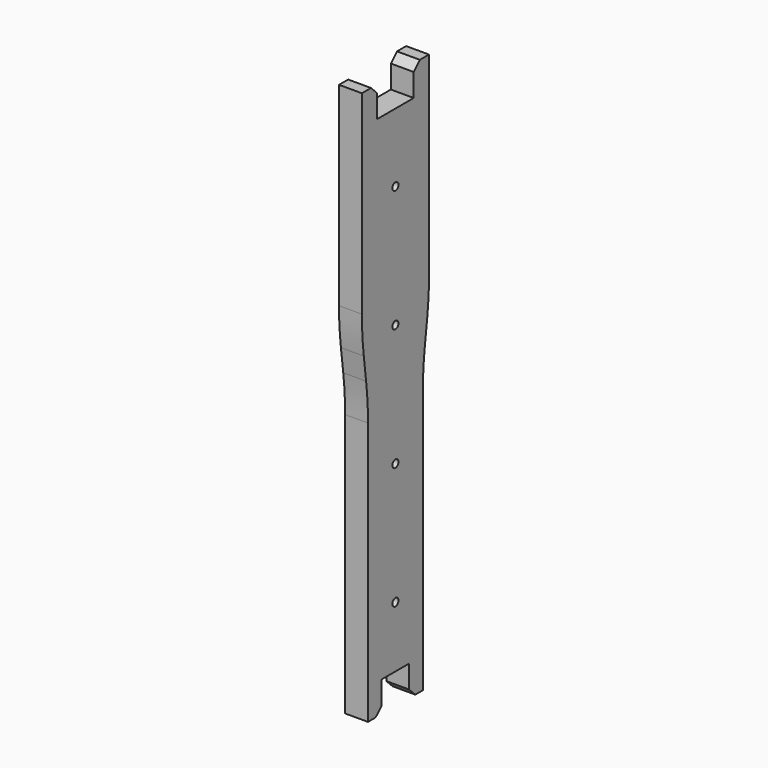
from build123d import *

# Parameters (mm, degrees)
F0_W     = 34.925
F0_H     = 231.775
F1_DEPTH = 9.525
F3_DEPTH = 9.525
F4_R     = 127
F5_W     = 19.05
F5_H     = 12.7
F5_W_2   = 14.2875
F6_DEPTH = 9.525
F7_SIZE  = 3.175
F9_D     = 3.175


# Not quite as in the source:
# - a pattern or mirror of a feature is missing from the dataset's text; its kind, count and spacing are read off the source's solid


with BuildPart() as f1:
    # F0 (on Right) → F1 (new body)
    with BuildSketch(Plane.YZ):
        with Locations((0, 115.8875)):
            Rectangle(F0_W, F0_H)
    extrude(amount=-F1_DEPTH)

    # F2 (on face) → F3 (cut, through all)
    with BuildSketch(Plane.YZ):
        Polygon((14.2875, 117.475), (14.2875, 0), (17.4625, 0), (17.4625, 142.875), align=None)
    f3 = extrude(amount=-F3_DEPTH, mode=Mode.SUBTRACT)

    # F3_copies: F3 across plane
    add(f3.mirror(Plane(origin=(0, 0, 0), x_dir=(0, 0, -1), z_dir=(0, -1, 0))), mode=Mode.SUBTRACT)

    # F4
    f4_edges = [f1.edges().sort_by_distance(p)[0] for p in [
        (-4.7625, 14.2875, 117.475),
        (-4.7625, 17.4625, 142.875),
        (-4.7625, -17.4625, 142.875),
        (-4.7625, -14.2875, 117.475),
    ]]
    fillet(f4_edges, radius=F4_R)

    # F5 (on face) → F6 (cut, through all)
    with BuildSketch(Plane.YZ):
        with Locations((0, 225.425)):
            Rectangle(F5_W, F5_H)
        with Locations((0, 6.35)):
            Rectangle(F5_W_2, F5_H)
    extrude(amount=-F6_DEPTH, mode=Mode.SUBTRACT)

    # F7
    f7_edges = [f1.edges().sort_by_distance(p)[0] for p in [
        (-4.7625, -9.525, 231.775),
        (-4.7625, 9.525, 231.775),
        (-4.7625, -7.14375, 0),
        (-4.7625, 7.14375, 0),
    ]]
    chamfer(f7_edges, length=F7_SIZE)

    # F9 (through all)
    with Locations(Plane.YZ):
        with Locations((0, 139.7), (0, 88.9), (0, 190.5), (0, 38.1)):
            Hole(F9_D / 2)


solid = f1.part
